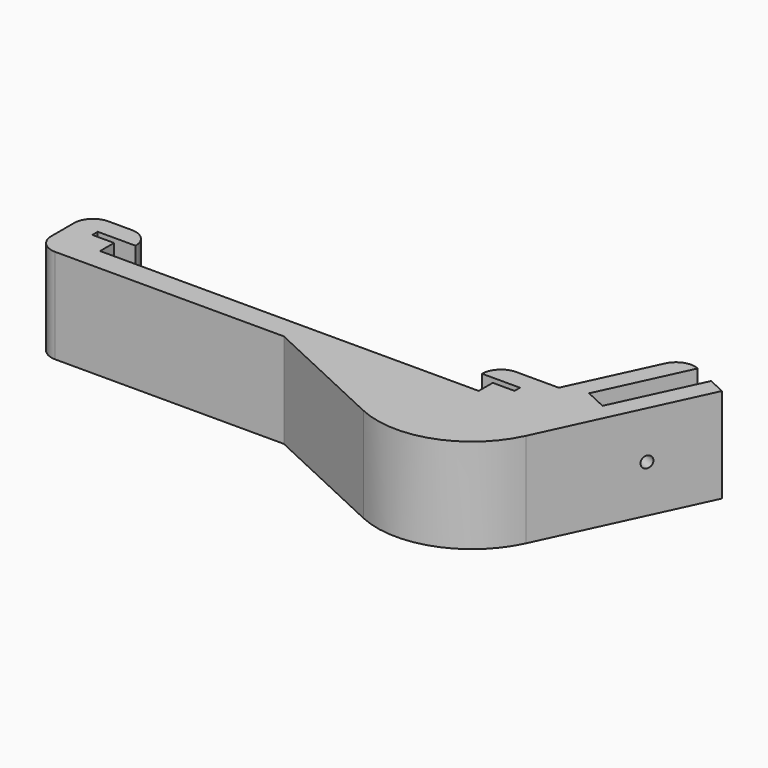
from build123d import *

# Parameters (mm, degrees)
F1_DEPTH = 25.4
F3_DEPTH = 25.4
F4_R     = 25.4
F5_R     = 5.07999
F6_R     = 1.524
F7_DEPTH = 25.4


# Not quite as in the source:
# - a fillet or chamfer is up to 0.001 mm smaller than in the source, because OpenCascade refuses the exact size


with BuildPart() as f1:
    # F0 (on Top) → F1 (new body)
    with BuildSketch(Plane.XY):
        Polygon((-46.482, 8.89), (-62.992, 8.89), (-62.992, -8.89), (62.992, -8.89), (62.992, 8.89), (46.482, 8.89), (46.482, 3.81), (56.642, 3.81), (56.642, 1.9812), (50.8, 1.9812), (50.8, -2.7178), (-50.8, -2.7178), (-50.8, 1.9812), (-56.642, 1.9812), (-56.642, 3.81), (-46.482, 3.81), align=None)
    extrude(amount=F1_DEPTH)

    # F2 (on face) → F3 (join)
    with BuildSketch(Plane.XY.offset(25.4)):
        Polygon((75.6565171085, 36.049144584), (62.992, 8.89), (62.992, -8.89), (3.4387046284, -8.89), (60.5084189693, -35.5020448459), (90.6196586724, 29.0717170827), (86.0156151143, 31.2186178523), (75.2811112661, 8.1984000616), (69.5260568184, 10.8820260237), (80.2605606666, 33.9022438144), align=None)
    extrude(amount=-F3_DEPTH)

    # F4
    f4_edges = [f1.edges().sort_by_distance(p)[0] for p in [
        (60.508419, -35.502045, 12.7),
    ]]
    fillet(f4_edges, radius=F4_R)

    # F5 (radius 5.08 in the source; OpenCascade refuses exactly that, so slightly less here)
    f5_edges = [f1.edges().sort_by_distance(p)[0] for p in [
        (-62.992, -8.89, 12.7),
        (-62.992, 8.89, 12.7),
        (75.656517, 36.049145, 12.7),
        (46.482, 8.89, 12.7),
        (-46.482, 8.89, 12.7),
    ]]
    fillet(f5_edges, radius=F5_R)

    # F6 (on face) → F7 (cut)
    with BuildSketch(Plane(origin=(48.336171005, -22.5395267055, 0), x_dir=(-0.4226182617, -0.906307787, 0), z_dir=(-0.906307787, 0.4226182617, 0))):
        with Locations((-47.1220459863, 12.7)):
            Circle(F6_R)
    extrude(amount=-F7_DEPTH, mode=Mode.SUBTRACT)


solid = f1.part
